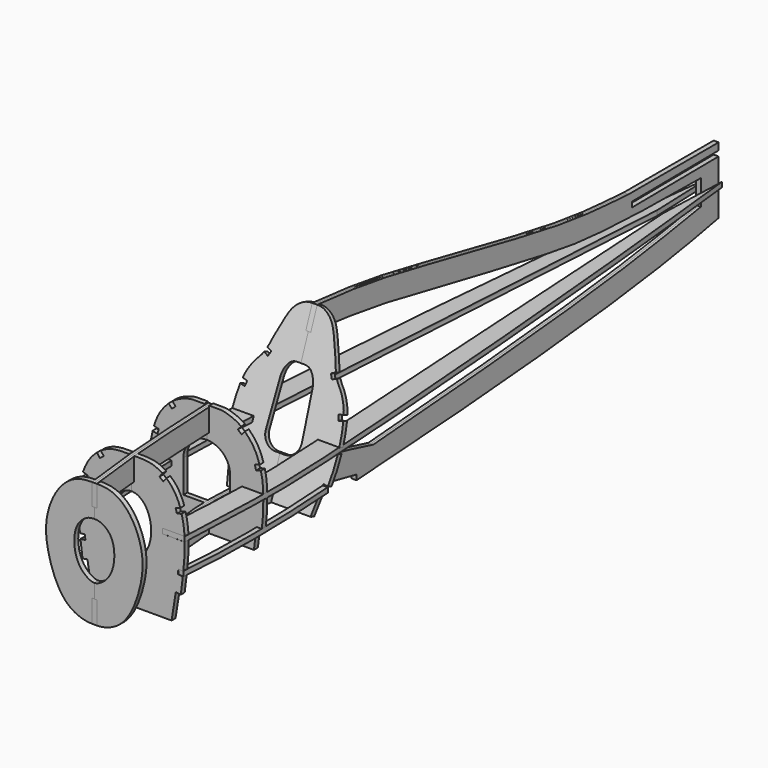
from build123d import *

# Parameters (mm, degrees)
F2_DEPTH  = 0.79375
F3_DEPTH  = 0.79375
F4_DEPTH  = 1.5875
F7_DEPTH  = 1.5875
F10_DEPTH = 1.5875
F16_DEPTH = 1.5875
F20_DEPTH = 1.5875
F24_DEPTH = 1.5875
F27_W     = 7.5223971916
F27_H     = 10.4603124782
F28_DEPTH = 1.5875
F29_W     = 7.5223971916
F29_H     = 10.5149038136
F30_DEPTH = 1.5875


with BuildPart() as f2:
    # F1 (on Right) → F2 (new body, symmetric)
    with BuildSketch(Plane.YZ):
        with BuildLine():
            Line((-46.8236642792, 32.4563067426), (-46.8236642792, 25.5481805935))
            add(Edge.make_bspline(
                [(-46.8236642792, 25.5481805935), (-41.1595846724, 26.129528907), (-28.3506810614, 27.4436731103), (-10.1500376549, 28.2173157507), (0, 28.6486744881)],
                knots=[0, 0, 0, 0, 0.4423238127, 1, 1, 1, 1], degree=3))
            Line((0, 28.6486744881), (0, 35.8860716224))
            add(Edge.make_bspline(
                [(-46.8236642792, 32.4563067426), (-37.0359072854, 33.6730802598), (-28.0089986254, 34.6104711154), (-9.0905161142, 35.5382358389), (0, 35.8860716224)],
                knots=[0, 0, 0, 0, 0.4683306715, 1, 1, 1, 1], degree=3))
        make_face()
    extrude(amount=F2_DEPTH, both=True)


with BuildPart() as f2b:
    # F1 (on Right) → F2, piece 2 (new body, symmetric)
    with BuildSketch(Plane.YZ):
        with BuildLine():
            Line((196.1769610643, 20.2713645995), (196.1769610643, 14.7688221186))
            Line((196.1769610643, 14.7688221186), (203.3381611109, 14.7688221186))
            Line((203.3381611109, 14.7688221186), (203.3381611109, 23.5155531693))
            Line((203.3381611109, 23.5155531693), (168.5410957955, 23.2019795107))
            Line((168.5410957955, 23.2019795107), (168.5259193182, 24.8861033469))
            Line((168.5259193182, 24.8861033469), (203.3381611109, 25.1998137683))
            Line((203.3381611109, 25.1998137683), (203.3381611109, 27.4956002831))
            Line((203.3381611109, 27.4956002831), (167.1288013458, 27.4956002831))
            add(Edge.make_bspline(
                [(41.8588146567, 47.1235960722), (48.785635612, 46.4818968428), (64.0962285717, 45.0635267466), (94.2588161112, 38.7779127007), (130.5031658843, 31.4983661174), (148.6901416918, 28.651994117), (161.0109340749, 27.8792867398), (167.1288013458, 27.4956002831)],
                knots=[0, 0, 0, 0, 0.1868112326, 0.4129153563, 0.6571956008, 0.8297810929, 1, 1, 1, 1], degree=3))
            Line((41.8588146567, 47.1235960722), (39.2708852887, 40.3623692691))
            add(Edge.make_bspline(
                [(196.1769610643, 20.2713645995), (189.0963530869, 20.306535579), (174.7183091676, 20.3778431614), (150.5345307383, 21.4209314002), (133.2832568356, 23.9448929276), (90.9187435491, 32.1674903363), (66.2529258562, 37.3287361638), (48.9414148033, 39.4045561552), (39.2708852887, 40.3623692691)],
                knots=[0, 0, 0, 0, 0.1527805236, 0.3102129977, 0.4504078664, 0.6630464807, 0.8309050847, 1, 1, 1, 1], degree=3))
        make_face()
    extrude(amount=F2_DEPTH, both=True)


with BuildPart() as f3:
    # F1 (on Right) → F3 (new body, symmetric)
    with BuildSketch(Plane.YZ):
        with BuildLine():
            Line((-46.8236642792, -0.4294639566), (-46.8236642792, -7.7078108206))
            add(Edge.make_bspline(
                [(-46.8236642792, -7.7078108206), (-44.9716311312, -7.9463409281), (-41.3971294994, -8.4067140373), (-36.6839390685, -8.4955020603), (-32.5049111076, -8.4824737125), (-30.2495229989, -8.475442417)],
                knots=[0, 0, 0, 0, 0.33107347, 0.6389856791, 1, 1, 1, 1], degree=3))
            Line((-30.2495229989, -8.475442417), (-30.2495229989, -6.6147418693))
            add(Edge.make_bspline(
                [(-30.2495229989, -6.6147418693), (-29.1059906606, -5.9954677379), (-26.3130781683, -4.482980159), (-17.5496624439, -1.5669324964), (-6.4277938524, 0.1512489332), (11.3783113795, 0.1864775748), (34.4905833836, -2.5017377687), (49.9292610921, -5.7593412283), (57.6750990003, -7.3937343314)],
                knots=[0, 0, 0, 0, 0.0926301832, 0.226235837, 0.376754002, 0.5644989401, 0.781501973, 1, 1, 1, 1], degree=3))
            Line((57.6750990003, -7.3937343314), (57.6750990003, -9.0407032639))
            add(Edge.make_bspline(
                [(57.6750990003, -9.0407032639), (72.3655662707, -8.1407784969), (102.6652601771, -6.2846465931), (152.7586556571, -1.91121059), (186.0417598816, 2.6261357632), (198.266712057, 5.0572639678), (203.3381611109, 6.0658031143)],
                knots=[0, 0, 0, 0, 0.2836465485, 0.5850326909, 0.8278532679, 1, 1, 1, 1], degree=3))
            Line((203.3381611109, 6.0658031143), (203.3381611109, 14.7688221186))
            Line((203.3381611109, 14.7688221186), (196.1769610643, 14.7688221186))
            Line((196.1769610643, 14.7688221186), (196.1769610643, 12.1344299987))
            add(Edge.make_bspline(
                [(64.4268617034, -1.6739845742), (80.4617044018, -0.514663314), (112.8876614178, 1.8297376919), (164.3828015949, 6.7636117523), (186.4738471886, 10.4953345824), (196.1769610643, 12.1344299987)],
                knots=[0, 0, 0, 0, 0.3542464769, 0.7163638116, 1, 1, 1, 1], degree=3))
            add(Edge.make_bspline(
                [(-33.4779247642, -1.2326592114), (-32.1150590653, -0.199306425), (-29.0529425571, 2.1224532528), (-21.1839670867, 5.5807445949), (-11.9399968538, 7.697589181), (0.8180338257, 8.7919052926), (22.0899054035, 7.3510190451), (44.2749221431, 3.5288611185), (57.8254528166, 0.0303730481), (64.4268617034, -1.6739845742)],
                knots=[0, 0, 0, 0, 0.0902278961, 0.2027260136, 0.3214153006, 0.4589577668, 0.6380858216, 0.8236863536, 1, 1, 1, 1], degree=3))
            add(Edge.make_bspline(
                [(-46.8236642792, -0.4294639566), (-45.370075456, -0.5399591212), (-42.4620279304, -0.7610155746), (-38.1091459028, -1.1973204539), (-35.0368323936, -1.2207638911), (-33.4779247642, -1.2326592114)],
                knots=[0, 0, 0, 0, 0.3298935707, 0.6599845615, 1, 1, 1, 1], degree=3))
        make_face()
    extrude(amount=F3_DEPTH, both=True)


with BuildPart() as f4:
    # F0 (on Front) → F4 (new body)
    with BuildSketch(Plane.XZ):
        with BuildLine():
            Line((0, 11.2188677477), (0, 8.4903640673))
            Line((0, 8.4903640673), (0.79375, 8.4903640673))
            Line((0.79375, 8.4903640673), (0.79375, 0))
            Line((0.79375, 0), (15.1883782819, 0))
            Line((15.1883782819, 0), (16.0051194319, 6.7865939066))
            Line((16.0051194319, 6.7865939066), (17.726002261, 6.7865939066))
            add(Edge.make_bspline(
                [(18.2002844859, 15.1531413235), (18.2136775269, 14.1190910319), (18.194366716, 11.1835910108), (17.908412647, 8.499059339), (17.726002261, 6.7865939066)],
                knots=[0.8087401121, 0.8087401121, 0.8087401121, 0.8087401121, 0.8779951267, 1, 1, 1, 1], degree=3))
            Line((18.2002844859, 15.1531413235), (11.3516710992, 15.1531413235))
            Line((11.3516710992, 15.1531413235), (11.3516710992, 16.7406413235))
            Line((11.3516710992, 16.7406413235), (18.1647018557, 16.7406413235))
            add(Edge.make_bspline(
                [(17.4163395053, 23.1857857778), (17.5174912527, 22.7821969276), (17.9732716618, 20.7615769396), (18.0902444126, 18.8747379916), (18.1558649582, 17.0246711386), (18.1647018557, 16.7406413235)],
                knots=[0.6129776399, 0.6129776399, 0.6129776399, 0.6129776399, 0.6404078661, 0.7526462558, 0.7725753276, 0.7725753276, 0.7725753276, 0.7725753276], degree=3))
            Line((17.4163395053, 23.1857857778), (15.8879962375, 22.7564571091))
            Line((15.8879962375, 22.7564571091), (15.4586675688, 24.2848003769))
            Line((15.4586675688, 24.2848003769), (16.9870108366, 24.7141290456))
            add(Edge.make_bspline(
                [(12.2650858571, 32.6132881156), (12.7850266157, 32.1184874663), (14.2502024826, 30.5241255773), (15.7254952267, 28.2750153382), (16.678888474, 25.7050245023), (16.9870108366, 24.7141290456)],
                knots=[0.3499477253, 0.3499477253, 0.3499477253, 0.3499477253, 0.4035594769, 0.5122409467, 0.578736948, 0.578736948, 0.578736948, 0.578736948], degree=3))
            Line((12.2650858571, 32.6132881156), (11.2337579345, 31.40642484))
            Line((11.2337579345, 31.40642484), (10.0268946589, 32.4377527625))
            Line((10.0268946589, 32.4377527625), (11.0582225814, 33.6446160382))
            add(Edge.make_bspline(
                [(0.79375, 36.2073231675), (2.0685647984, 36.2524724397), (4.4340427184, 36.3362490059), (7.0634913284, 35.7434751761), (9.5406888585, 34.7331355752), (10.858207727, 33.7962516073), (11.0582225814, 33.6446160382)],
                knots=[0, 0, 0, 0, 0.101378177, 0.1881119043, 0.2914647684, 0.3103534159, 0.3103534159, 0.3103534159, 0.3103534159], degree=3))
            Line((0.79375, 36.2073231675), (0.79375, 28.6390148103))
            Line((0.79375, 28.6390148103), (0, 28.6390148103))
            Line((0, 28.6390148103), (0, 26.2636621309))
            ThreePointArc((0, 26.2636621309), (7.5223971916, 18.7412649393), (0, 11.2188677477))
        make_face()
    extrude(amount=F4_DEPTH)


with BuildPart() as f7:
    # F6 (on offset) → F7 (new body)
    with BuildSketch(Plane.XZ.offset(30.226)):
        with BuildLine():
            Line((0.79375, 34.2662739642), (0.79375, 27.080743573))
            Line((0.79375, 27.080743573), (0, 27.080743573))
            Line((0, 27.080743573), (0, 23.9719673991))
            add(Edge.make_bspline(
                [(0, 5.4802009836), (6.2890359261, 5.4802009836), (6.2890359261, 14.7260841914), (6.2890359261, 23.9719673991), (0, 23.9719673991)],
                knots=[3.1415926536, 3.1415926536, 3.1415926536, 4.7123889804, 4.7123889804, 6.2831853072, 6.2831853072, 6.2831853072], degree=2, weights=[1, 0.7071067812, 1, 0.7071067812, 1]))
            Line((0, 5.4802009836), (0, 1.0978171226))
            Line((0, 1.0978171226), (0.79375, 1.0978171226))
            Line((0.79375, 1.0978171206), (0.79375, -6.6020031638))
            Line((0.79375, -6.6020031638), (0.79375, -8.475442417))
            Line((0.79375, -8.475442417), (12.8569891676, -8.475442417))
            Line((12.8569891676, -8.475442417), (14.2150307074, 0.0549967481))
            Line((14.2150307074, 0.0549967481), (15.8109679196, -0.1990756375))
            add(Edge.make_bspline(
                [(16.4624029105, 5.1250159629), (16.2639480286, 3.3707543649), (16.0374579741, 1.5858393637), (15.8109679196, -0.1990756375)],
                knots=[0.8937781715, 0.8937781715, 0.8937781715, 0.8937781715, 1, 1, 1, 1], degree=3))
            Line((16.4624029105, 5.1250159629), (14.8841571726, 5.296178578))
            Line((14.8841571726, 5.296178578), (15.0553197877, 6.8744243159))
            Line((15.0553197877, 6.8744243159), (16.6335655256, 6.7032617008))
            add(Edge.make_bspline(
                [(17.0898779619, 15.1428457856), (17.1160158545, 13.7611636438), (17.0361732912, 11.0449713179), (16.7817407359, 8.137883879), (16.6335655256, 6.7032617008)],
                knots=[0.6800875178, 0.6800875178, 0.6800875178, 0.6800875178, 0.7738034873, 0.8617376688, 0.8617376688, 0.8617376688, 0.8617376688], degree=3))
            Line((17.0898779619, 15.1428457856), (9.8791308701, 15.1428457856))
            Line((9.8791308701, 15.1428457856), (9.8791308701, 16.7303457856))
            Line((9.8791308701, 16.7303457856), (17.0286404344, 16.7303457856))
            add(Edge.make_bspline(
                [(16.10538846, 22.8231577141), (16.3484483908, 21.8855771041), (16.7565802141, 19.8329027504), (16.9644058217, 17.8174138076), (17.0286404344, 16.7303457856)],
                knots=[0.505674191, 0.505674191, 0.505674191, 0.505674191, 0.5697408951, 0.644038483, 0.644038483, 0.644038483, 0.644038483], degree=3))
            Line((16.10538846, 22.8231577141), (14.582687067, 22.3742293036))
            Line((14.582687067, 22.3742293036), (14.1337586565, 23.8969306966))
            Line((14.1337586565, 23.8969306966), (15.6564600495, 24.3458591071))
            add(Edge.make_bspline(
                [(11.1753923015, 31.3026653837), (12.0865671016, 30.5195753234), (13.9616615657, 28.4410092797), (15.1542806841, 25.8535889893), (15.6564600495, 24.3458591071)],
                knots=[0.2817222159, 0.2817222159, 0.2817222159, 0.2817222159, 0.365345082, 0.4706508285, 0.4706508285, 0.4706508285, 0.4706508285], degree=3))
            Line((11.1753923015, 31.3026653837), (10.2129515412, 30.0401821034))
            Line((10.2129515412, 30.0401821034), (8.9504682609, 31.0026228637))
            Line((8.9504682609, 31.0026228637), (9.9129090212, 32.265106144))
            add(Edge.make_bspline(
                [(0.79375, 34.2662739642), (3.001426626, 34.3004534818), (6.1046512696, 34.3484979826), (9.0919655919, 32.8164715237), (9.9129090212, 32.265106144)],
                knots=[0, 0, 0, 0, 0.1738982042, 0.2444403253, 0.2444403253, 0.2444403253, 0.2444403253], degree=3))
        make_face()
    extrude(amount=F7_DEPTH)


with BuildPart() as f10:
    # F9 (on offset) → F10 (new body)
    with BuildSketch(Plane(origin=(0, 20.7777218793, -7.9528875777), x_dir=(1, 0, 0), z_dir=(0, -0.9339248582, 0.3574693822))):
        with BuildLine():
            Line((0.79375, 58.9731423949), (0.79375, 51.7335590991))
            Line((0.79375, 51.7335590991), (0, 51.7335590991))
            Line((0, 51.7335590991), (0, 43.4074495028))
            Line((0, 43.4074495028), (0.8790718432, 43.4074495028))
            add(Edge.make_bspline(
                [(0.8790718432, 43.4074495028), (1.5628326309, 43.4074495028), (3.1603944865, 43.2575983813), (4.8272738651, 40.7476716313), (5.159674395, 39.010753566), (5.1879687235, 38.3687503636)],
                knots=[0, 0, 0, 0, 0.3106885067, 0.6719339518, 1, 1, 1, 1], degree=3))
            Line((5.1879687235, 38.3687503636), (5.8073685504, 24.3144612759))
            ThreePointArc((5.8073685504, 24.3144612759), (4.6136893834, 21.1399696454), (1.4948329774, 19.807677716))
            Line((1.4948329774, 19.807677716), (0, 19.807677716))
            Line((0, 19.807677716), (0, 15.3808808914))
            Line((0, 15.3808808914), (0.79375, 15.3808808914))
            Line((0.79375, 15.3808808914), (0.79375, 7.1204841439))
            Line((0.79375, 7.1204841439), (13.4574016556, 7.1204841439))
            Line((13.4574016556, 7.1204841439), (15.0594273582, 16.2323229015))
            Line((15.0594273582, 16.2323229015), (16.4975232102, 15.9794796962))
            add(Edge.make_bspline(
                [(17.2422063972, 24.7808646917), (17.2424670438, 24.1282429179), (17.1845195396, 20.8906827506), (16.8030479622, 18.1636159339), (16.4975232102, 15.9794796962)],
                knots=[0.8602449692, 0.8602449692, 0.8602449692, 0.8602449692, 0.888068744, 1, 1, 1, 1], degree=3))
            Line((17.2422063972, 24.7808646917), (10.3519679978, 24.7808646917))
            Line((10.3519679978, 24.7808646917), (10.3519679978, 26.3683646917))
            Line((10.3519679978, 26.3683646917), (17.2191175665, 26.3683646917))
            add(Edge.make_bspline(
                [(16.5884550605, 33.1432352445), (16.688239157, 32.583277465), (16.9886704778, 30.592152987), (17.1698362951, 28.1097424243), (17.2191175665, 26.3683646917)],
                knots=[0.7320507483, 0.7320507483, 0.7320507483, 0.7320507483, 0.7641486185, 0.8378171192, 0.8378171192, 0.8378171192, 0.8378171192], degree=3))
            Line((16.5884550605, 33.1432352445), (15.0344315046, 32.8189405674))
            Line((15.0344315046, 32.8189405674), (14.7101368275, 34.3729641234))
            Line((14.7101368275, 34.3729641234), (16.2641603834, 34.6972588004))
            add(Edge.make_bspline(
                [(11.7236059231, 42.8760865198), (11.8495395076, 42.6408505648), (12.450124144, 41.5999095335), (13.5401083742, 40.6609557524), (15.14481508, 37.9573567031), (15.8259638311, 36.3383991492), (16.1705364929, 35.0825147891), (16.2641603834, 34.6972588004)],
                knots=[0.4539618645, 0.4539618645, 0.4539618645, 0.4539618645, 0.4711185153, 0.5343000767, 0.6074650647, 0.673610014, 0.6998139612, 0.6998139612, 0.6998139612, 0.6998139612], degree=3))
            Line((11.7236059231, 42.8760865198), (10.2903259023, 42.1935437504))
            Line((10.2903259023, 42.1935437504), (9.6077831329, 43.6268237712))
            Line((9.6077831329, 43.6268237712), (11.0410631537, 44.3093665405))
            add(Edge.make_bspline(
                [(0.79375, 58.9731423949), (2.0075370558, 58.9693933725), (3.5835661324, 58.548321753), (6.3332655899, 56.4925919481), (8.1476605754, 52.5115828088), (10.3083718172, 46.5779650071), (10.4775900685, 45.7094828296), (10.8685937888, 44.7112814683), (11.0410631537, 44.3093665405)],
                knots=[0, 0, 0, 0, 0.0719694858, 0.1462839647, 0.2386337193, 0.3432596265, 0.3917406615, 0.4205191889, 0.4205191889, 0.4205191889, 0.4205191889], degree=3))
        make_face()
    extrude(amount=-F10_DEPTH)


with BuildPart() as f11_1:
    # F11: instance of F7
    add(f7.part.mirror(Plane.YZ))


with BuildPart() as f12_1:
    # F12: instance of F4
    add(f4.part.mirror(Plane.YZ))

    # F29 (on face) → F30 (cut, through all)
    with BuildSketch(Plane(origin=(0, 0, 0), x_dir=(-1, 0, 0), z_dir=(0, 1, 0))):
        with Locations((3.7611985958, 13.4838130325)):
            Rectangle(F29_W, F29_H)
    extrude(amount=-F30_DEPTH, mode=Mode.SUBTRACT)


with BuildPart() as f13_1:
    # F13: instance of F10
    add(f10.part.mirror(Plane.YZ))


with BuildPart() as f16:
    # F15 (on offset) → F16 (new body)
    with BuildSketch(Plane.XY.offset(15.1531413235)):
        with BuildLine():
            Line((9.8791308701, -31.8135), (17.0898779619, -31.8135))
            add(Edge.make_bspline(
                [(17.0898779619, -31.8135), (17.5670497389, -21.2496455852), (18.5732280436, 0.0729737444), (17.5284794441, 33.5241484413), (9.7849182785, 133.9276134968), (1.9591038581, 203.2154202461)],
                knots=[0, 0, 0, 0, 0.2264245152, 0.4565318679, 1, 1, 1, 1], degree=3))
            Line((1.9591038581, 203.2154202461), (1.105046249, 180.920034647))
            add(Edge.make_bspline(
                [(10.3519679978, 29.7339292797), (8.6206441637, 60.5673886101), (4.8628452064, 120.7437116285), (1.105046249, 180.920034647)],
                knots=[0.4741906827, 0.4741906827, 0.4741906827, 0.4741906827, 1, 1, 1, 1], degree=3))
            add(Edge.make_bspline(
                [(11.3516710992, -1.5875), (11.5077018944, 7.7553671875), (11.1394639038, 15.7092722454), (10.3519679978, 29.7339292797)],
                knots=[0.2350253246, 0.2350253246, 0.2350253246, 0.2350253246, 0.4741906827, 0.4741906827, 0.4741906827, 0.4741906827], degree=3))
            add(Edge.make_bspline(
                [(9.8791308701, -31.8135), (10.5387360601, -21.291069494), (11.1983412501, -10.7686389879), (11.3516710992, -1.5875)],
                knots=[0, 0, 0, 0, 0.2350253246, 0.2350253246, 0.2350253246, 0.2350253246], degree=3))
        make_face()
    extrude(amount=F16_DEPTH)


with BuildPart() as f17_1:
    # F17: instance of F16
    add(f16.part.mirror(Plane.YZ))


with BuildPart() as f20:
    # F19 (on offset) → F20 (new body)
    with BuildSketch(Plane(origin=(0, 0, 6.7865939066), x_dir=(1, 0, 0), z_dir=(0, 0, -1))):
        with BuildLine():
            add(Edge.make_bspline(
                [(16.6335655246, 31.8135), (17.5424389601, 21.649949725), (18.1088081111, 1.669498343), (17.1585582772, -17.2125607573), (16.4975232102, -26.4898966139)],
                knots=[0, 0, 0, 0, 0.509178227, 1, 1, 1, 1], degree=3))
            Line((16.6335655246, 31.8135), (15.0523751627, 31.6721023705))
            add(Edge.make_bspline(
                [(15.0523751627, 31.6721023705), (15.4958131516, 26.7133214037), (16.0859263139, 16.7854623207), (16.2391603466, 2.0706047653), (15.8205466286, -12.2455465916), (15.249938978, -21.6628433943), (14.9140377553, -26.3770690274)],
                knots=[0, 0, 0, 0, 0.25, 0.5, 0.75, 1, 1, 1, 1], degree=3))
            Line((14.9140377553, -26.3770690274), (16.4975232102, -26.4898966139))
        make_face()
    extrude(amount=F20_DEPTH)


with BuildPart() as f24:
    # F23 (on 3pt) → F24 (new body)
    with BuildSketch(Plane.XZ.offset(46.8236642792)):
        with BuildLine():
            Line((0.79375, 32.4563067426), (0.79375, 25.5481805935))
            Line((0.79375, 25.5481805935), (0, 25.5481805935))
            Line((0, 25.5481805935), (0, 22.2406145185))
            add(Edge.make_bspline(
                [(0, 22.2406145185), (0.7735663094, 22.2274642438), (2.3846546595, 22.0806827485), (5.581402943, 19.4841535869), (6.5966116402, 15.1825420533), (6.3612213987, 10.6207333162), (4.3954795926, 6.14489333), (1.2288880534, 4.1206236929), (0, 4.1196071543)],
                knots=[0, 0, 0, 0, 0.126426089, 0.288831167, 0.4620327224, 0.6391987649, 0.8236897904, 1, 1, 1, 1], degree=3))
            Line((0, 4.1196071543), (0, -0.4294639566))
            Line((0, -0.4294639566), (0.79375, -0.4294639566))
            Line((0.79375, -0.4294639566), (0.79375, -7.7078108206))
            add(Edge.make_bspline(
                [(0.79375, 32.4563067426), (4.1698156856, 32.4705690145), (8.0403515856, 31.1050161562), (12.7880980717, 25.9658804434), (15.8877799911, 17.6250688683), (15.4409577833, 8.1467063546), (10.3681913327, -5.6657786673), (3.075538436, -7.7242301777), (0.79375, -7.7078108206)],
                knots=[0, 0, 0, 0, 0.1516568374, 0.2928941942, 0.455140681, 0.6286103082, 0.8370349306, 1, 1, 1, 1], degree=3))
        make_face()
    extrude(amount=-F24_DEPTH)


with BuildPart() as f25_1:
    # F25: instance of F24
    add(f24.part.mirror(Plane.YZ))


with BuildPart() as f4_1:
    add(f4.part)

    # F27 (on face) → F28 (cut, through all)
    with BuildSketch(Plane(origin=(0, 0, 0), x_dir=(-1, 0, 0), z_dir=(0, 1, 0))):
        with Locations((-3.7611985958, 13.5111087002)):
            Rectangle(F27_W, F27_H)
    extrude(amount=-F28_DEPTH, mode=Mode.SUBTRACT)


solid = Compound([f2.part, f2b.part, f3.part, f7.part, f10.part, f11_1.part, f12_1.part, f13_1.part, f16.part, f17_1.part, f20.part, f24.part, f25_1.part, f4_1.part])
